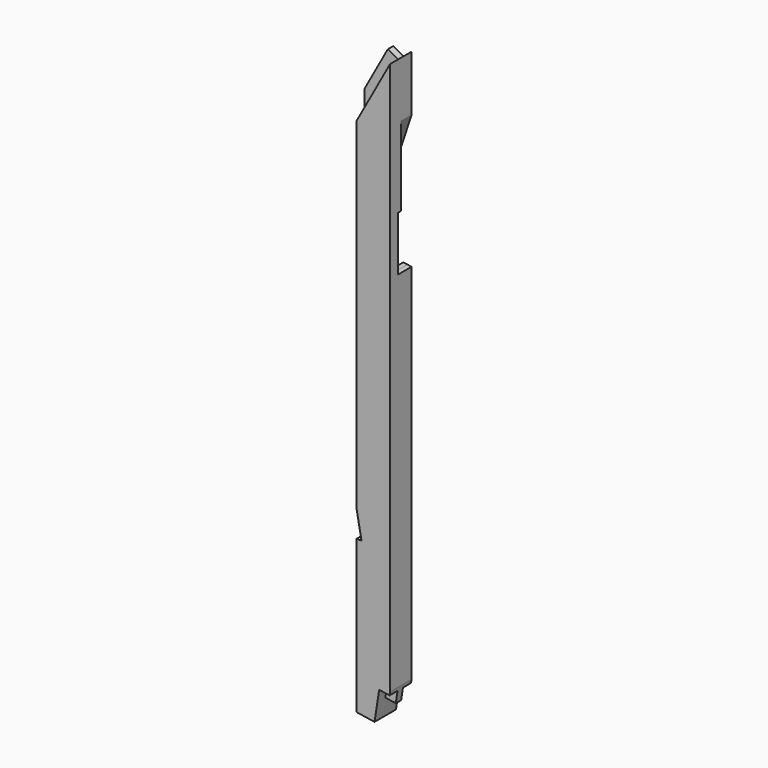
from build123d import *

# Parameters (mm, degrees)
F1_DEPTH = 101.6
F2_DEPTH = 25.4
F4_DEPTH = 127
F5_DEPTH = 101.6
F6_W     = 50.8
F6_H     = 609.6
F7_DEPTH = 114.3


# Not quite as in the source:
# - a feature names something its author has since deleted; it is built from what else it names


with BuildPart() as f1:
    # F0 (on Front) → F1 (new body, symmetric)
    with BuildSketch(Plane.XZ):
        Polygon((48.5735566343, -2087.3053811025), (-127, -2059.9159062675), (-127, -2316.988), (9.4230761062, -2338.2699998726), (30.9558403967, -2200.239459549), (44.6585085815, -2112.4018429795), align=None)
        Polygon((123.0849519472, -2124.6363681445), (127, -2099.5399062675), (48.5735566343, -2087.3053811025), (44.6585085815, -2112.4018429795), align=None)
        Polygon((127, -2099.5399062675), (127, -1584.5717697842), (48.5735566343, -2087.3053811025), align=None)
        Polygon((127, 2083.5330486298), (-127, 1621.3110685349), (-127, -959.054172039), (-88.9, -1162.254172039), (-127, -1162.254172039), (-127, -2059.9159062675), (48.5735566343, -2087.3053811025), (127, -1584.5717697842), (127, 1383.5908232688), align=None)
    extrude(amount=F1_DEPTH, both=True)

    # F0 (on Front) → F2 (join, symmetric)
    with BuildSketch(Plane.XZ):
        Polygon((109.3822837623, -2212.4739847141), (123.0849519472, -2124.6363681445), (44.6585085815, -2112.4018429795), (30.9558403967, -2200.239459549), align=None)
        Polygon((49.0886035459, 2126.3468817047), (-127, 1805.9058462593), (-127, 1621.3110685349), (127, 2083.5330486298), align=None)
    extrude(amount=F2_DEPTH, both=True)

    # F3 (on face) → F4 (cut)
    with BuildSketch(Plane(origin=(0, 101.6, 0), x_dir=(-1, 0, 0), z_dir=(0, 1, 0))):
        Polygon((-124.6851625392, 841.1452440828), (-65.1155717719, 659.9737911019), (127, 689.9630318555), (127, 890.3500338664), (125.3471307259, 895.3658269662), (-127, 855.9744398599), align=None)
        Polygon((127, 895.6238398599), (125.3471307259, 895.3658269662), (127, 890.3500338664), align=None)
        Polygon((-127, 1061.6352478643), (-127, 855.9744398599), (125.3471307259, 895.3658269662), (60.8907531403, 1090.9649944295), align=None)
        Polygon((60.8907531403, 1090.9649944295), (125.3471307259, 895.3658269662), (127, 895.6238398599), (127, 1101.2846478643), align=None)
        Polygon((-124.6851625392, 841.1452440828), (-95.6600158458, 655.2058033819), (-65.1155717719, 659.9737911019), align=None)
        Polygon((-127, 848.1854547136), (-127, 650.3136318555), (-95.6600158458, 655.2058033819), (-124.6851625392, 841.1452440828), align=None)
        Polygon((-127, 855.9744398599), (-127, 848.1854547136), (-124.6851625392, 841.1452440828), align=None)
    extrude(amount=-F4_DEPTH, mode=Mode.SUBTRACT)

    # F3 (on face) → F5 (cut)
    with BuildSketch(Plane(origin=(0, 101.6, 0), x_dir=(-1, 0, 0), z_dir=(0, 1, 0))):
        Polygon((127, 650.3136318555), (-61.9392891755, 650.3136318555), (127, 75.6847800506), align=None)
        Polygon((-65.1155717719, 659.9737911019), (-61.9392891755, 650.3136318555), (127, 650.3136318555), (127, 689.9630318555), align=None)
        Polygon((-127, 1661.1378192902), (-127, 1061.6352478643), (60.8907531403, 1090.9649944295), align=None)
    extrude(amount=-F5_DEPTH, mode=Mode.SUBTRACT)

    # F6 (on face) → F7 (cut)
    with BuildSketch(Plane(origin=(-127, 0, 0), x_dir=(0, -1, 0), z_dir=(-1, 0, 0))):
        with Locations((0, -1467.054172039)):
            Rectangle(F6_W, F6_H)
    extrude(amount=-F7_DEPTH, mode=Mode.SUBTRACT)


solid = f1.part
